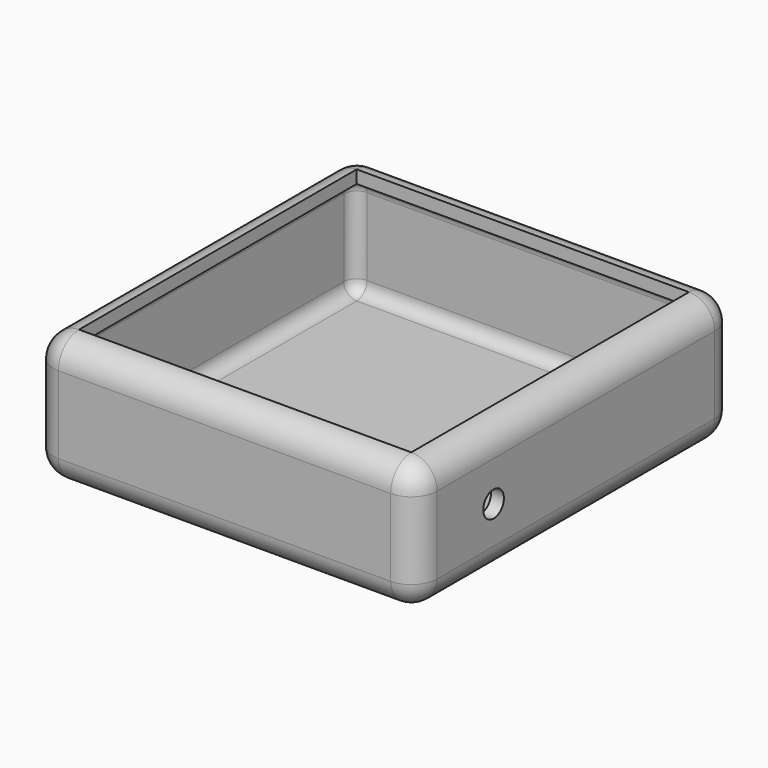
from build123d import *

# Parameters (mm, degrees)
F0_W     = 74.4920149446
F0_H     = 77.3611664772
F1_DEPTH = 25
F2_R     = 5
F3_T     = -2.5
F5_D     = 5
F5_DEPTH = 12
F5_TIP   = 1.5021515476


# Not quite as in the source:
# - a shell that OpenCascade refuses in one call is made with other operations: the cavity is built on its own and cut out


with BuildPart() as f1:
    # F0 (on Top) → F1 (new body)
    with BuildSketch(Plane.XY):
        with Locations((-7.9336054623, -1.4722160995)):
            Rectangle(F0_W, F0_H)
    extrude(amount=F1_DEPTH)

    # F2
    f2_edges = [f1.edges().sort_by_distance(p)[0] for p in [
        (29.312402, -40.152799, 12.5),
        (29.312402, -1.472216, 25),
        (-7.933605, -40.152799, 25),
        (-45.179613, -1.472216, 25),
        (-7.933605, 37.208367, 25),
        (29.312402, -1.472216, 0),
        (-7.933605, -40.152799, 0),
        (29.312402, 37.208367, 12.5),
        (-45.179613, -40.152799, 12.5),
        (-45.179613, 37.208367, 12.5),
        (-45.179613, -1.472216, 0),
        (-7.933605, 37.208367, 0),
    ]]
    fillet(f2_edges, radius=F2_R)

    # F3: a shell. OpenCascade refuses it in one call, so the cavity is built on its own and cut out:
    # the body offset inwards by the wall thickness, plus a prism from it out through each open face.
    f3_core = offset(f1.part, amount=F3_T, mode=Mode.PRIVATE)
    f3_exits = [f3_core.faces().sort_by_distance(p)[0] for p in [
        (-7.933605, -1.472216, 22.5),
    ]]
    add(f3_core, mode=Mode.SUBTRACT)
    extrude(f3_exits, amount=-F3_T, mode=Mode.SUBTRACT)

    # F5
    with Locations(Plane.YZ.offset(29.31240201)):
        with Locations((-21.4438159019, 12.2315008193)):
            Hole(F5_D / 2, depth=F5_DEPTH)
            with Locations((0, 0, -(F5_DEPTH + F5_TIP / 2))):  # 118° drill point
                Cone(0, F5_D / 2, F5_TIP, mode=Mode.SUBTRACT)


solid = f1.part
